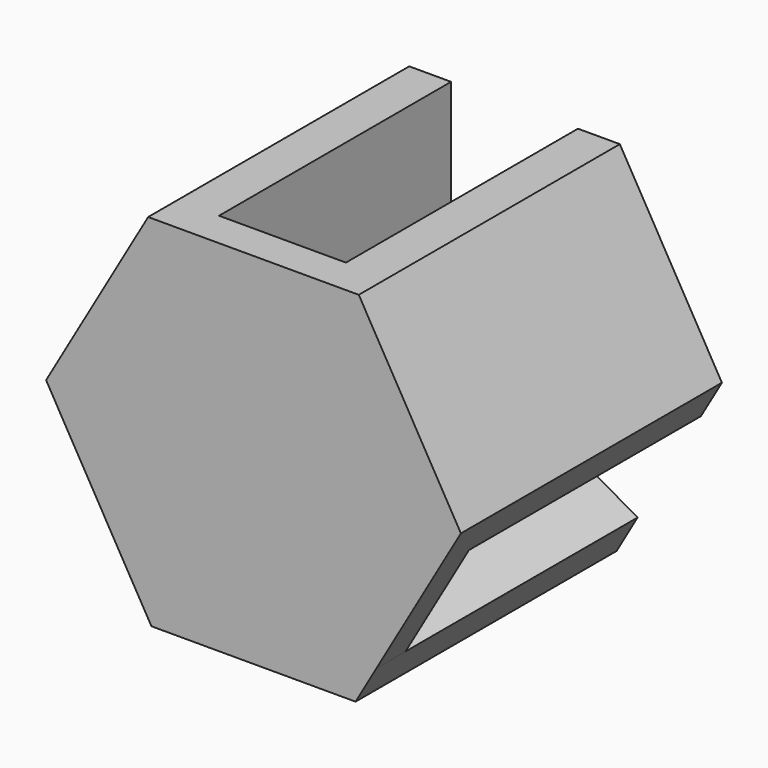
from build123d import *

# Parameters (mm, degrees)
F2_DEPTH = 3.175
F3_DEPTH = 25.4


# Not quite as in the source:
# - a feature names something its author has since deleted; it is built from what else it names


with BuildPart() as f2:
    # F1 (on Front) → F2 (new body)
    with BuildSketch(Plane.XZ):
        Polygon((-18.1618179038, 0.1631008549), (-16.3287307991, -3.0118991451), (-6.1622247723, 2.8577358462), (-6.1622247723, 3.5577621311), (-5.5559842263, 3.9077752735), (-5.5559842263, 15.6470452561), (-9.2221584356, 15.6470452561), align=None)
        Polygon((6.1622247723, 2.8577358462), (16.3287307991, -3.0118991451), (18.1618179038, 0.1631008549), (9.2221584356, 15.6470452561), (5.5559842263, 15.6470452561), (5.5559842263, 3.9077752735), (6.1622247723, 3.5577621311), align=None)
        Polygon((-0.606240546, -6.7655111197), (-10.7727465728, -12.635146111), (-8.9396594682, -15.810146111), (8.9396594682, -15.810146111), (10.7727465728, -12.635146111), (0.606240546, -6.7655111197), (0, -7.1155242622), align=None)
        Polygon((5.5559842263, 3.2077489886), (6.1622247723, 2.8577358462), (6.1622247723, 3.5577621311), (5.5559842263, 3.9077752735), align=None)
        Polygon((-6.1622247723, 3.5577621311), (-6.1622247723, 2.8577358462), (-5.5559842263, 3.2077489886), (-5.5559842263, 3.9077752735), align=None)
        Polygon((0, -6.4154979773), (-0.606240546, -6.7655111197), (0, -7.1155242622), (0.606240546, -6.7655111197), align=None)
        Polygon((-6.1622247723, -3.5577621311), (-0.606240546, -6.7655111197), (0, -6.4154979773), (0.606240546, -6.7655111197), (6.1622247723, -3.5577621311), (6.1622247723, 2.8577358462), (5.5559842263, 3.2077489886), (5.5559842263, 3.9077752735), (0, 7.1155242622), (-5.5559842263, 3.9077752735), (-5.5559842263, 3.2077489886), (-6.1622247723, 2.8577358462), align=None)
        Polygon((5.5559842263, 15.6470452561), (-5.5559842263, 15.6470452561), (-5.5559842263, 3.9077752735), (0, 7.1155242622), (5.5559842263, 3.9077752735), align=None)
        Polygon((-16.3287307991, -3.0118991451), (-10.7727465728, -12.635146111), (-0.606240546, -6.7655111197), (-6.1622247723, -3.5577621311), (-6.1622247723, 2.8577358462), align=None)
        Polygon((0.606240546, -6.7655111197), (10.7727465728, -12.635146111), (16.3287307991, -3.0118991451), (6.1622247723, 2.8577358462), (6.1622247723, -3.5577621311), align=None)
    extrude(amount=F2_DEPTH)

    # F1 (on Front) → F3 (join)
    with BuildSketch(Plane.XZ):
        Polygon((-18.1618179038, 0.1631008549), (-16.3287307991, -3.0118991451), (-6.1622247723, 2.8577358462), (-6.1622247723, 3.5577621311), (-5.5559842263, 3.9077752735), (-5.5559842263, 15.6470452561), (-9.2221584356, 15.6470452561), align=None)
        Polygon((-0.606240546, -6.7655111197), (-10.7727465728, -12.635146111), (-8.9396594682, -15.810146111), (8.9396594682, -15.810146111), (10.7727465728, -12.635146111), (0.606240546, -6.7655111197), (0, -7.1155242622), align=None)
        Polygon((6.1622247723, 2.8577358462), (16.3287307991, -3.0118991451), (18.1618179038, 0.1631008549), (9.2221584356, 15.6470452561), (5.5559842263, 15.6470452561), (5.5559842263, 3.9077752735), (6.1622247723, 3.5577621311), align=None)
        Polygon((-6.1622247723, -3.5577621311), (-0.606240546, -6.7655111197), (0, -6.4154979773), (0.606240546, -6.7655111197), (6.1622247723, -3.5577621311), (6.1622247723, 2.8577358462), (5.5559842263, 3.2077489886), (5.5559842263, 3.9077752735), (0, 7.1155242622), (-5.5559842263, 3.9077752735), (-5.5559842263, 3.2077489886), (-6.1622247723, 2.8577358462), align=None)
        Polygon((5.5559842263, 3.2077489886), (6.1622247723, 2.8577358462), (6.1622247723, 3.5577621311), (5.5559842263, 3.9077752735), align=None)
        Polygon((0, -6.4154979773), (-0.606240546, -6.7655111197), (0, -7.1155242622), (0.606240546, -6.7655111197), align=None)
        Polygon((-6.1622247723, 3.5577621311), (-6.1622247723, 2.8577358462), (-5.5559842263, 3.2077489886), (-5.5559842263, 3.9077752735), align=None)
    extrude(amount=-F3_DEPTH)


solid = f2.part
